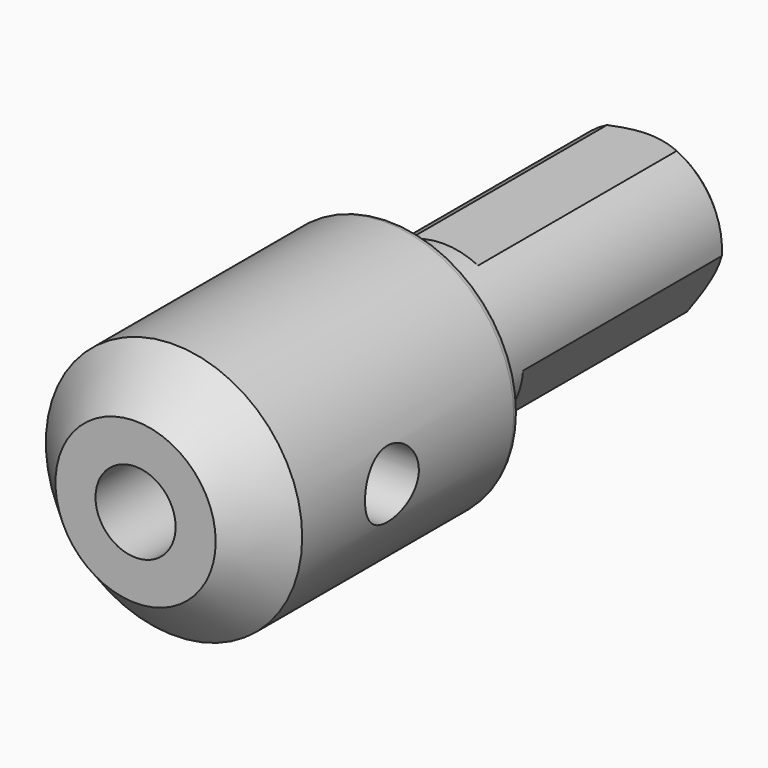
from build123d import *

# Parameters (mm, degrees)
F0_R            = 8
F1_DEPTH        = 20
F2_R            = 5
F3_DEPTH        = 20
F5_DEPTH        = 16
F5_COPIES_COUNT = 3
F6_SIZE         = 0.49999
F7_R            = 0.5
F9_D            = 5
F9_DEPTH        = 14
F9_TIP          = 1.5021515476
F10_R           = 2.1
F11_DEPTH       = 8.25
F12_SIZE        = 3


# Not quite as in the source:
# - a fillet or chamfer is up to 0.001 mm smaller than in the source, because OpenCascade refuses the exact size
# - a pattern or mirror of a feature is missing from the dataset's text; its kind, count and spacing are read off the source's solid


with BuildPart() as f1:
    # F0 (on Front) → F1 (new body)
    with BuildSketch(Plane.XZ):
        Circle(F0_R)
    extrude(amount=-F1_DEPTH)

    # F2 (on face) → F3 (join)
    with BuildSketch(Plane(origin=(0, 20, 0), x_dir=(-1, 0, 0), z_dir=(0, 1, 0))):
        Circle(F2_R)
    extrude(amount=F3_DEPTH)

    # F4 (on face) → F5 (cut)
    with BuildSketch(Plane(origin=(0, 40, 0), x_dir=(-1, 0, 0), z_dir=(0, 1, 0))):
        with BuildLine():
            ThreePointArc((2.1794494718, 4.5), (0, 5), (-2.1794494718, 4.5))
            Line((-2.1794494718, 4.5), (2.1794494718, 4.5))
        make_face()
    f5 = extrude(amount=-F5_DEPTH, mode=Mode.SUBTRACT)

    # F5_copies: F5 ×3 about axis
    f5_copies_axis = Axis((0, 0, 0), (0, 1, 0))
    for i in range(1, F5_COPIES_COUNT):
        add(f5.rotate(f5_copies_axis, i * 360 / F5_COPIES_COUNT), mode=Mode.SUBTRACT)

    # F6 (size 0.5 in the source; OpenCascade refuses exactly that, so slightly less here)
    f6_edges = [f1.edges().sort_by_distance(p)[0] for p in [
        (4.330127, 40, 2.5),
        (-4.996709, 40, -0.18139),
        (0, 40, -5),
        (-4.236582, 40, 2.655443),
    ]]
    chamfer(f6_edges, length=F6_SIZE)

    # F7
    f7_edges = [f1.edges().sort_by_distance(p)[0] for p in [
        (-8, 20, 0),
        (5, 20, 0),
    ]]
    fillet(f7_edges, radius=F7_R)

    # F9
    with Locations(Plane.XZ):
        with Locations((0, 0)):
            Hole(F9_D / 2, depth=F9_DEPTH)
            with Locations((0, 0, -(F9_DEPTH + F9_TIP / 2))):  # 118° drill point
                Cone(0, F9_D / 2, F9_TIP, mode=Mode.SUBTRACT)

    # F10 (on Right) → F11 (cut, symmetric)
    with BuildSketch(Plane.YZ):
        with Locations((10, 0)):
            Circle(F10_R)
    extrude(amount=F11_DEPTH, both=True, mode=Mode.SUBTRACT)

    # F12
    f12_edges = [f1.edges().sort_by_distance(p)[0] for p in [
        (-8, 0, 0),
    ]]
    chamfer(f12_edges, length=F12_SIZE)


solid = f1.part
